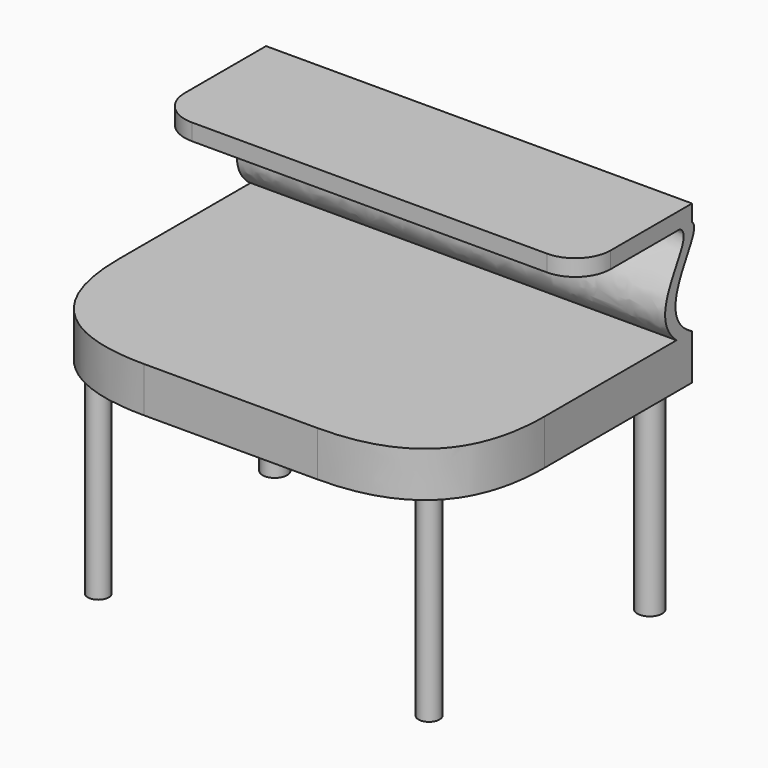
from build123d import *

# Parameters (mm, degrees)
F0_W        = 76.5841603279
F0_H        = 55.8080822229
F2_DEPTH    = 8.128
F4_DEPTH    = 2.9718
F6_DEPTH    = 76.9874
F7_T1_DEPTH = 121.5718952959
F8_R        = 2.2102169693
F8_R_2      = 1.8884160903
F9_DEPTH    = 35.814


# Not quite as in the source:
# - a fillet or chamfer that OpenCascade refuses, or shapes differently, is made with other operations: its cross-section is extruded or revolved along the edge and cut away or added


with BuildPart() as f2:
    # F0 (on Top) → F2 (new body)
    with BuildSketch(Plane.XY):
        with Locations((-38.292080164, 27.9040411115)):
            Rectangle(F0_W, F0_H)
    extrude(amount=F2_DEPTH)



with BuildPart() as f4:
    # F3 (on offset) → F4 (new body)
    with BuildSketch(Plane.XY.offset(25.4)):
        with BuildLine():
            ThreePointArc((-6.35, 31.1775822192), (-1.8598719395, 33.0374541587), (0, 37.5275822192))
            Line((0, 37.5275822192), (0, 55.8080822229))
            Line((0, 55.8080822229), (-76.5841603279, 55.8080822229))
            Line((-76.5841603279, 55.8080822229), (-76.5841603279, 37.5275822192))
            ThreePointArc((-76.5841603279, 37.5275822192), (-74.7242883884, 33.0374541587), (-70.2341603279, 31.1775822192))
            Line((-70.2341603279, 31.1775822192), (-6.35, 31.1775822192))
        make_face()
    extrude(amount=F4_DEPTH)


with BuildPart() as f2_1:
    add(f2.part)

    add(f4.part)  # F6 merges F4
    # F5 (on Right) → F6 (join)
    with BuildSketch(Plane.YZ):
        with BuildLine():
            add(Edge.make_bspline(
                [(55.8080822229, 25.4), (58.8490366814, 23.136356831), (46.0850115883, 13.5771517675), (55.8080822229, 8.128)],
                knots=[0, 0, 0, 0, 17.272, 17.272, 17.272, 17.272], degree=3))
            Line((55.8080822229, 25.4), (53.1005598605, 25.4))
            add(Edge.make_bspline(
                [(53.1005598605, 25.4), (57.1686353537, 22.7699241637), (44.6180654452, 14.8183666988), (52.3269809783, 8.128)],
                knots=[0, 0, 0, 0, 17.2893148588, 17.2893148588, 17.2893148588, 17.2893148588], degree=3))
            Line((52.3269809783, 8.128), (55.8080822229, 8.128))
        make_face()
    extrude(amount=-F6_DEPTH)

    # F7: fillet of radius 22.6887790592 on 2 edges, made by hand

    # F7_s2 → F7_t1 (cut)
    with BuildSketch(Plane.XY.offset(-56.721947648)):
        with BuildLine():
            add(Edge.make_bspline(
                [(-53.8953812687, 0), (-76.5841603279, 0), (-76.5841603279, 22.6887790592)],
                knots=[0, 0, 0, 1, 1, 1], degree=2, weights=[1, 1, 1]))
            Line((-76.5841603279, 22.6887790592), (-76.5841603279, 0))
            Line((-76.5841603279, 0), (-53.8953812687, 0))
        make_face()
        with BuildLine():
            add(Edge.make_bspline(
                [(0, 22.6887790592), (0, 0), (-22.6887790592, 0)],
                knots=[0, 0, 0, 1, 1, 1], degree=2, weights=[1, 1, 1]))
            Line((-22.6887790592, 0), (0, 0))
            Line((0, 0), (0, 22.6887790592))
        make_face()
    extrude(amount=F7_T1_DEPTH, mode=Mode.SUBTRACT)

    # F8 (on face) → F9 (join)
    with BuildSketch(Plane(origin=(0, 0, 0), x_dir=(1, 0, 0), z_dir=(0, 0, -1))):
        with Locations((-71.9979479909, -52.0507059991)):
            Circle(F8_R)
        with Locations((-68.019554019, -7.4042403139)):
            Circle(F8_R_2)
        with Locations((-4.586212337, -52.0507059991)):
            Circle(F8_R)
        with Locations((-8.5646063089, -7.4042403139)):
            Circle(F8_R_2)
    extrude(amount=F9_DEPTH)


solid = f2_1.part
